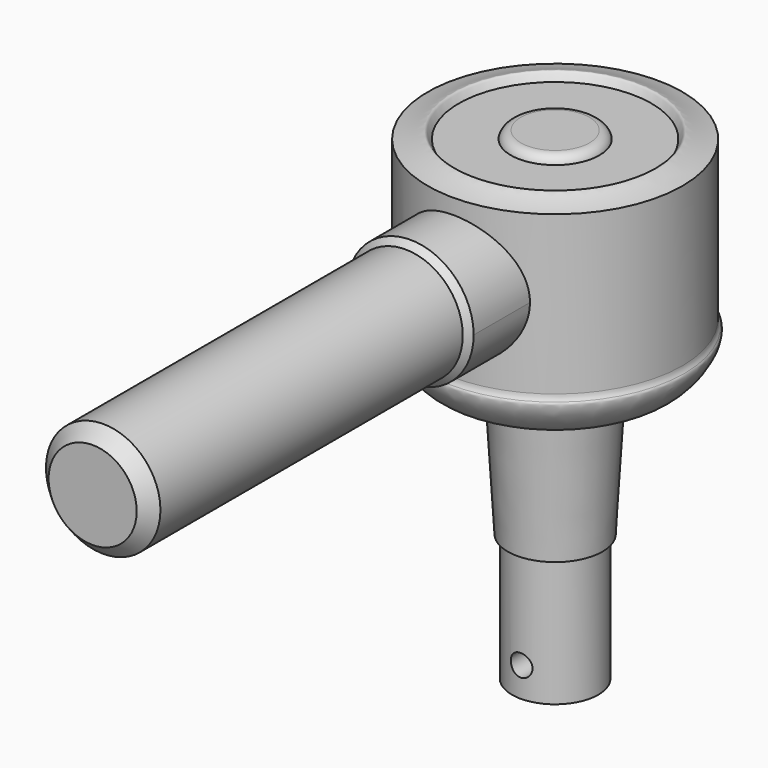
from build123d import *

# Parameters (mm, degrees)
F2_R        = 1.778
F3_DEPTH    = 12.7
F5_DEPTH    = 31.75
F6_R        = 9.3599
F7_DEPTH    = 62.7888
F8_S5_R     = 9.3599
F8_T6_DEPTH = 16


# Not quite as in the source:
# - a fillet or chamfer that OpenCascade refuses, or shapes differently, is made with other operations: its cross-section is extruded or revolved along the edge and cut away or added


with BuildPart() as f1:
    # F0 (on Front) → F1 (revolve)
    with BuildSketch(Plane.XZ):
        with BuildLine():
            Line((6.35, 58.166), (0, 58.166))
            Line((0, 58.166), (0, 30.226))
            Line((0, 30.226), (0, 19.685))
            Line((0, 19.685), (0, 0))
            Line((0, 0), (0, -20.828))
            Line((0, -20.828), (7.0612, -20.828))
            Line((7.0612, -20.828), (7.0612, 0))
            Line((7.0612, 0), (7.747, 0))
            Line((7.747, 0), (8.90905, 19.685))
            add(Edge.make_bspline(
                [(8.90905, 19.685), (11.7912068963, 27.2870212793), (16.1954839903, 19.0053529362), (22.480616346, 29.8321191221), (20.828, 30.226)],
                knots=[0, 0, 0, 0, 0.5235722787, 1, 1, 1, 1], degree=3))
            Line((20.828, 30.226), (20.828, 56.896))
            add(Edge.make_bspline(
                [(15.748, 56.896), (16.993034631, 59.2658407986), (16.2821896374, 57.6469525695), (20.828, 56.896)],
                knots=[0, 0, 0, 0, 5.08, 5.08, 5.08, 5.08], degree=3))
            Line((15.748, 56.896), (7.239, 56.896))
            Line((7.239, 56.896), (7.239, 58.166))
            Line((7.239, 58.166), (6.35, 58.166))
        make_face()
    revolve(axis=Axis((0, 0, -8.4981196864), (0, 0, -1)))

    # F2 (on Front) → F3 (cut, symmetric)
    with BuildSketch(Plane.XZ):
        with Locations((0, -16.002)):
            Circle(F2_R)
    extrude(amount=F3_DEPTH, both=True, mode=Mode.SUBTRACT)

    # F4 (on Front) → F5 (join)
    with BuildSketch(Plane.XZ):
        with BuildLine():
            ThreePointArc((0, 33.7185), (7.3189087387, 36.7500912613), (10.3505, 44.069))
            ThreePointArc((10.3505, 44.069), (-7.3189087387, 51.3879087387), (0, 33.7185))
        make_face()
    extrude(amount=F5_DEPTH)

    # F6 (on face) → F7 (join)
    with BuildSketch(Plane.XZ.offset(31.75)):
        with Locations((0, 44.069)):
            Circle(F6_R)
    extrude(amount=F7_DEPTH)

    # F8: chamfer of 2.159 on 2 edges, made by hand


with BuildPart() as f8_tool2:
    # F8_s3 → F8_t4 (revolve)
    with BuildSketch(Plane.YZ):
        Polygon((-29.591, 33.7185), (-31.75, 35.8775), (-31.75, 33.7185), align=None)
    revolve(axis=Axis((0, -31.75, 44.069), (0, 1, 0)))

    # F8_s5 → F8_t6 (cut, symmetric)
    with BuildSketch(Plane.XZ.offset(30.7)):
        with Locations((0, 44.069)):
            Circle(F8_S5_R)
    extrude(amount=F8_T6_DEPTH, both=True, mode=Mode.SUBTRACT)


with BuildPart() as f1_1:
    add(f1.part)

    # F8_t1: cut F8_tool2
    add(f8_tool2.part, mode=Mode.SUBTRACT)

    # F8_s7 → F8_t8 (revolve, cut)
    with BuildSketch(Plane.XY.offset(44.069)):
        Polygon((9.3599, -92.3798), (7.2009, -94.5388), (9.3599, -94.5388), align=None)
    revolve(axis=Axis((0, -94.5388, 44.069), (0, -1, 0)), mode=Mode.SUBTRACT)

    # F9: fillet of radius 1.651 on 2 edges, made by hand

    # F9_s1 → F9_t2 (revolve, cut)
    with BuildSketch(Plane.XZ):
        with BuildLine():
            ThreePointArc((7.239, 56.896), (6.6564696827, 57.8101509565), (5.6325629486, 58.166))
            Line((5.6325629486, 58.166), (5.6325629486, 58.19902))
            Line((5.6325629486, 58.19902), (7.239, 58.19902))
            Line((7.239, 58.19902), (7.27202, 58.166))
            ThreePointArc((7.27202, 58.166), (7.27202, 57.531), (7.271128741, 56.90362))
            Line((7.271128741, 56.90362), (7.239, 56.896))
        make_face()
    revolve(axis=Axis((0, 0, 58.166), (0, 0, -1)), mode=Mode.SUBTRACT)

    # F9_s3 → F9_t4 (revolve)
    with BuildSketch(Plane.XZ):
        with BuildLine():
            ThreePointArc((21.1597456512, 30.0175911775), (20.9131312427, 30.4869361434), (20.828, 31.010248703))
            Line((20.828, 31.010248703), (20.79498, 31.010248703))
            Line((20.79498, 31.010248703), (20.79498, 30.226))
            Line((20.79498, 30.226), (20.8203445184, 30.1938796949))
            ThreePointArc((20.8203445184, 30.1938796949), (20.9949538129, 30.1235602191), (21.1333605642, 29.997738027))
            Line((21.1333605642, 29.997738027), (21.1597456512, 30.0175911775))
        make_face()
    revolve(axis=Axis((0, 0, 30.226), (0, 0, -1)))


solid = f1_1.part
